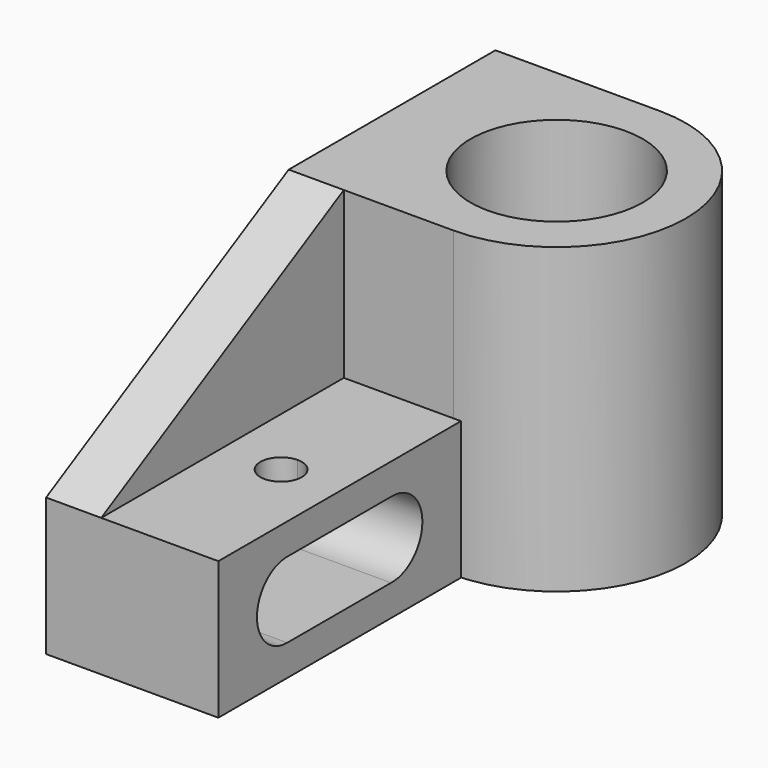
from build123d import *

# Parameters (mm, degrees)
F0_R     = 25
F1_DEPTH = 88
F2_W     = 88
F2_H     = 40
F3_DEPTH = 50
F5_DEPTH = 16
F7_DEPTH = 9.008194986


with BuildPart() as f1:
    # F0 (on Top) → F1 (new body)
    with BuildSketch(Plane.XY):
        with BuildLine():
            Line((0, 75), (0, 0))
            Line((0, 0), (47.7671325207, 0))
            ThreePointArc((47.7671325207, 0), (85.2671325207, 37.5), (47.7671325207, 75))
            Line((47.7671325207, 75), (0, 75))
        make_face()
        with Locations((47.7671325207, 37.5)):
            Circle(F0_R, mode=Mode.SUBTRACT)
    extrude(amount=F1_DEPTH)

    # F2 (on Right) → F3 (join)
    with BuildSketch(Plane.YZ):
        with Locations((-44, 20)):
            Rectangle(F2_W, F2_H)
        with BuildLine():
            ThreePointArc((-63.4935666774, 30.9889213272), (-63.0031659942, 30.9999995444), (-62.5127590152, 30.989203621))
            Line((-62.5127590152, 30.989203621), (-25.0031659942, 30.9999995444))
            ThreePointArc((-25.0031659942, 30.9999995444), (-14.0013797727, 19.8257786016), (-25.3515634815, 9.0056194755))
            Line((-25.3515634815, 9.0056194755), (-62.9983580838, 9.0000001225))
            ThreePointArc((-62.9983580838, 9.0000001225), (-62.9991790419, 9.0000000306), (-63, 9))
            ThreePointArc((-63, 9), (-73.997229983, 19.7531545007), (-63.4935666774, 30.9889213272))
        make_face(mode=Mode.SUBTRACT)
    extrude(amount=F3_DEPTH)

    # F4 (on Right) → F5 (join)
    with BuildSketch(Plane.YZ):
        Polygon((-88, 40), (0, 40), (0, 88), align=None)
    extrude(amount=F5_DEPTH)

    # F6 (on face) → F7 (cut, through all)
    with BuildSketch(Plane.XY.offset(40)):
        with BuildLine():
            ThreePointArc((39, -44), (37.2426406871, -39.7573593129), (33, -38))
            ThreePointArc((33, -38), (28.7573593129, -48.2426406871), (39, -44))
        make_face()
    extrude(amount=-F7_DEPTH, mode=Mode.SUBTRACT)


solid = f1.part
